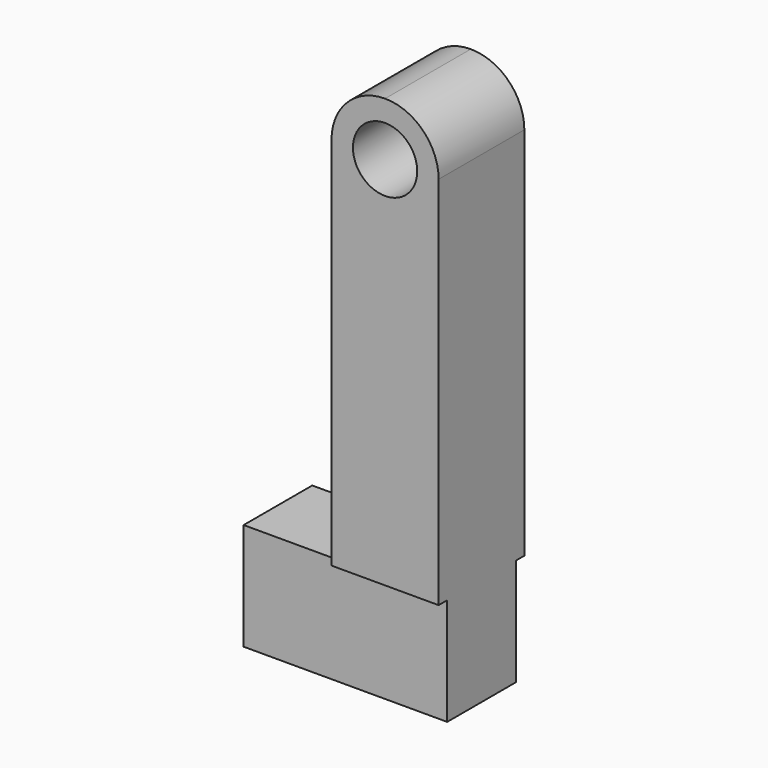
from build123d import *

# Parameters (mm, degrees)
F0_W     = 5
F0_H     = 5
F1_DEPTH = 5
F2_D     = 3
F3_R     = 2.49999
F4_W     = 4
F4_H     = 5
F5_DEPTH = 9.5


# Not quite as in the source:
# - a fillet or chamfer is up to 0.001 mm smaller than in the source, because OpenCascade refuses the exact size


with BuildPart() as f1:
    # F0 (on Front) → F1 (new body)
    with BuildSketch(Plane.XZ):
        Polygon((4.8, 5), (9.8, 5), (9.8, 15), (9.8, 20), (4.8, 20), align=None)
        with Locations((7.3, 22.5)):
            Rectangle(F0_W, F0_H)
    extrude(amount=F1_DEPTH)

    # F2 (through all)
    with Locations(Plane(origin=(0, 0, 0), x_dir=(1, 0, 0), z_dir=(0, 1, 0))):
        with Locations((7.3, -22.5)):
            Hole(F2_D / 2)

    # F3 (radius 2.5 in the source; OpenCascade refuses exactly that, so slightly less here)
    f3_edges = [f1.edges().sort_by_distance(p)[0] for p in [
        (4.8, -2.5, 25),
        (9.8, -2.5, 25),
    ]]
    fillet(f3_edges, radius=F3_R)

    # F4 (on face) → F5 (join)
    with BuildSketch(Plane.YZ.offset(9.8)):
        with Locations((-2.5, 2.5)):
            Rectangle(F4_W, F4_H)
    extrude(amount=-F5_DEPTH)


solid = f1.part
